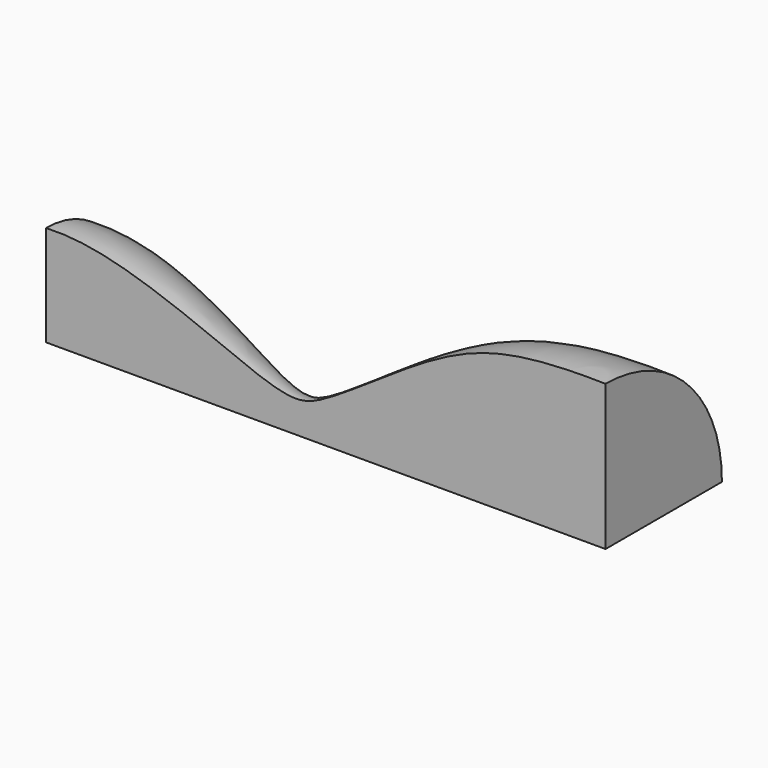
from build123d import *

# Parameters (mm, degrees)
F1_ANGLE = 90


with BuildPart() as f1:
    # F0 (on Top) → F1 (revolve)
    with BuildSketch(Plane.XY):
        with BuildLine():
            add(Edge.make_bspline(
                [(0, 18), (4.369673031, 18.200553342), (13.7879697958, 16.8138650428), (30.5549450805, 10.2926748944), (43.5549683653, 4.7106670496), (50.3110572543, 6.9945874011), (66.4756233338, 18.7583350429), (80.6912774182, 25.7060429411), (93.4094842344, 26.1386142265), (100, 26)],
                knots=[0, 0, 0, 0, 0.1366196461, 0.2965833322, 0.4315071917, 0.5259494023, 0.6890114049, 0.8389412371, 1, 1, 1, 1], degree=3))
            Line((0, 18), (0, 0))
            Line((0, 0), (100, 0))
            Line((100, 0), (100, 26))
        make_face()
    revolve(axis=Axis((50, 0, 0), (1, 0, 0)), revolution_arc=F1_ANGLE)


solid = f1.part
